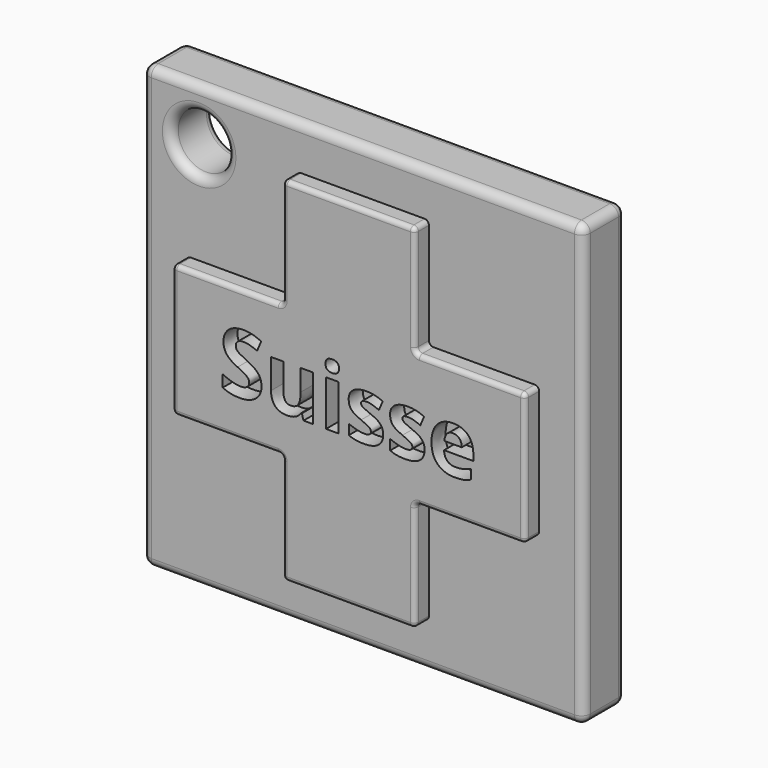
from build123d import *

# Parameters (mm, degrees)
F0_W         = 15
F0_H         = 15
F0_W_2       = 12.5
F0_H_2       = 12.5
F1_DEPTH     = 5
F0_W_3       = 50
F0_H_3       = 50
F2_DEPTH     = 3
F3_TEXT_SIZE = 8.7625932388
F4_DEPTH     = 1.5
F5_R         = 3.1663942209
F6_DEPTH     = 25
F7_R         = 1
F8_R         = 0.5
F9_TEXT_SIZE = 9.4466700426
F10_DEPTH    = 2


# Not quite as in the source:
# - Text() gives the source's letters only with a copy of the font that has no kerning and outlines rounded to 1/6400 em; it was checked with that copy


with BuildPart() as f1:
    # F0 (on Front) → F1 (new body, symmetric)
    with BuildSketch(Plane.XZ):
        Rectangle(F0_W, F0_H)
        with Locations((-13.75, 0)):
            Rectangle(F0_W_2, F0_H)
        with Locations((13.75, 0)):
            Rectangle(F0_W_2, F0_H)
        with Locations((0, -13.75)):
            Rectangle(F0_W, F0_H_2)
        with Locations((0, 13.75)):
            Rectangle(F0_W, F0_H_2)
    extrude(amount=F1_DEPTH, both=True)

    # F0 (on Front) → F2 (join, symmetric)
    with BuildSketch(Plane.XZ):
        Rectangle(F0_W_3, F0_H_3)
        Polygon((7.5, -7.5), (7.5, -20), (-7.5, -20), (-7.5, -7.5), (-20, -7.5), (-20, 7.5), (-7.5, 7.5), (-7.5, 20), (7.5, 20), (7.5, 7.5), (20, 7.5), (20, -7.5), align=None, mode=Mode.SUBTRACT)
    extrude(amount=F2_DEPTH, both=True)

    # F3 (on face) → F4 (join, symmetric)
    with BuildSketch(Plane(origin=(0, 5, 0), x_dir=(-1, 0, 0), z_dir=(0, 1, 0))):
        with Locations((-9.4429447781, -2.8210578021)):
            Text('Joao', F3_TEXT_SIZE, font='Open Sans', font_style=FontStyle.BOLD, text_align=(TextAlign.LEFT, TextAlign.BOTTOM))
    extrude(amount=F4_DEPTH, both=True)

    # F5 (on face) → F6 (cut)
    with BuildSketch(Plane(origin=(0, 3, 0), x_dir=(-1, 0, 0), z_dir=(0, 1, 0))):
        with Locations((18.5694117099, 19.1044788808)):
            Circle(F5_R)
    extrude(amount=-F6_DEPTH, mode=Mode.SUBTRACT)

    # F7
    f7_edges = [f1.edges().sort_by_distance(p)[0] for p in [
        (0, -3, -25),
        (25, -3, 0),
        (-25, -3, 0),
        (0, -3, 25),
        (25, 0, 25),
        (25, 0, -25),
        (-25, 0, -25),
        (-25, 0, 25),
        (0, 3, 25),
        (-25, 3, 0),
        (25, 3, 0),
        (0, 3, -25),
        (-15.403017, 3, 19.104479),
        (-15.403017, -3, 19.104479),
    ]]
    fillet(f7_edges, radius=F7_R)

    # F8
    f8_edges = [f1.edges().sort_by_distance(p)[0] for p in [
        (-20, -5, 0),
        (-20, -4, 7.5),
        (-13.75, -5, 7.5),
        (-13.75, -5, -7.5),
        (-7.5, -5, -13.75),
        (-7.5, -4, -7.5),
        (-20, -4, -7.5),
        (0, -5, -20),
        (-7.5, -4, -20),
        (7.5, -5, -13.75),
        (13.75, -5, -7.5),
        (7.5, -4, -7.5),
        (7.5, -4, -20),
        (20, -4, -7.5),
        (20, -5, 0),
        (20, -4, 7.5),
        (13.75, -5, 7.5),
        (7.5, -4, 7.5),
        (7.5, -5, 13.75),
        (7.5, -4, 20),
        (0, -5, 20),
        (-7.5, -5, 13.75),
        (-7.5, -4, 20),
        (-7.5, -4, 7.5),
        (7.5, 5, 13.75),
        (-7.5, 5, 13.75),
        (0, 5, 20),
        (13.75, 5, 7.5),
        (20, 5, 0),
        (13.75, 5, -7.5),
        (7.5, 5, -13.75),
        (0, 5, -20),
        (-7.5, 4, -7.5),
        (-13.75, 5, -7.5),
        (-7.5, 5, -13.75),
        (-20, 5, 0),
        (-13.75, 5, 7.5),
        (-7.5, 4, 7.5),
        (-20, 4, 7.5),
        (-20, 4, -7.5),
        (-7.5, 4, -20),
        (7.5, 4, -20),
        (7.5, 4, -7.5),
        (20, 4, -7.5),
        (20, 4, 7.5),
        (7.5, 4, 7.5),
        (7.5, 3, 13.75),
        (7.5, 4, 20),
        (-7.5, 4, 20),
        (0, 3, 20),
        (-7.5, 3, 13.75),
    ]]
    fillet(f8_edges, radius=F8_R)

    # F9 (on face) → F10 (cut)
    with BuildSketch(Plane.XZ.offset(5)):
        with Locations((-14.7245214321, -3.2881887164)):
            Text('Suisse', F9_TEXT_SIZE, font='Open Sans', font_style=FontStyle.BOLD, text_align=(TextAlign.LEFT, TextAlign.BOTTOM))
    extrude(amount=-F10_DEPTH, mode=Mode.SUBTRACT)


solid = f1.part
